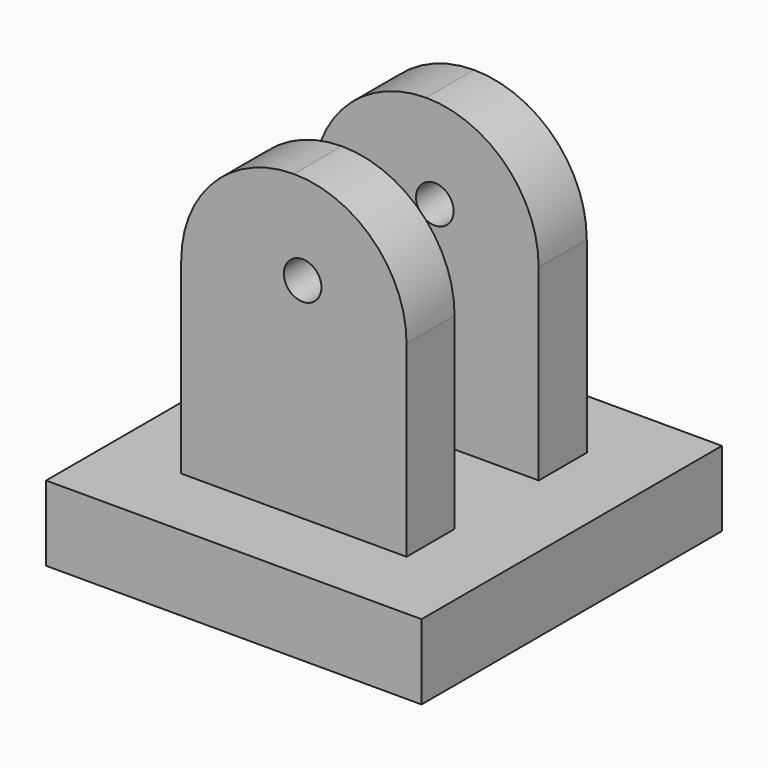
from build123d import *

# Parameters (mm, degrees)
F0_W     = 50
F0_H     = 50
F1_DEPTH = 10
F2_W     = 30
F2_H     = 8
F3_DEPTH = 40
F4_W     = 30
F4_H     = 8
F5_DEPTH = 40
F6_R     = 14.99999
F7_R     = 14.99999
F9_D     = 5


# Not quite as in the source:
# - a fillet or chamfer is up to 0.001 mm smaller than in the source, because OpenCascade refuses the exact size


with BuildPart() as f1:
    # F0 (on Top) → F1 (new body)
    with BuildSketch(Plane.XY):
        Rectangle(F0_W, F0_H)
    extrude(amount=F1_DEPTH)

    # F2 (on face) → F3 (join)
    with BuildSketch(Plane.XY.offset(10)):
        with Locations((0, -11)):
            Rectangle(F2_W, F2_H)
    extrude(amount=F3_DEPTH)

    # F4 (on face) → F5 (join)
    with BuildSketch(Plane.XY.offset(10)):
        with Locations((0, 11)):
            Rectangle(F4_W, F4_H)
    extrude(amount=F5_DEPTH)

    # F6 (radius 15 in the source; OpenCascade refuses exactly that, so slightly less here)
    f6_edges = [f1.edges().sort_by_distance(p)[0] for p in [
        (-15, -11, 50),
        (15, -11, 50),
    ]]
    fillet(f6_edges, radius=F6_R)

    # F7 (radius 15 in the source; OpenCascade refuses exactly that, so slightly less here)
    f7_edges = [f1.edges().sort_by_distance(p)[0] for p in [
        (15, 11, 50),
        (-15, 11, 50),
    ]]
    fillet(f7_edges, radius=F7_R)

    # F9 (through all)
    with Locations(Plane.XZ.offset(15)):
        with Locations((1.1680303141, 37.8934629261)):
            Hole(F9_D / 2)


solid = f1.part
